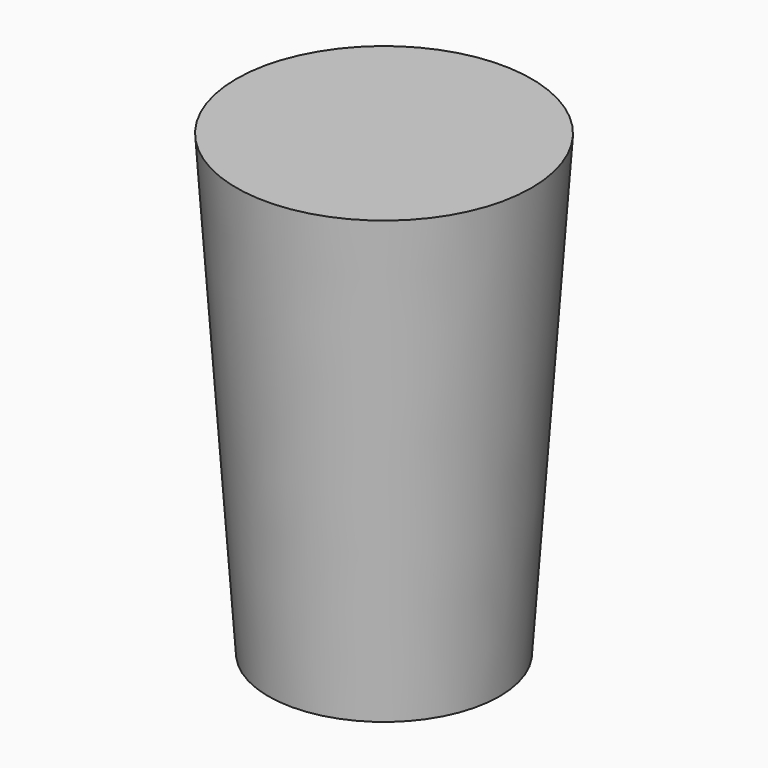
from build123d import *

# Parameters (mm, degrees)
F0_R     = 50.4693117614
F1_DEPTH = 200
F1_TAPER = -4


with BuildPart() as f1:
    # F0 (on Top) → F1 (new body)
    with BuildSketch(Plane.XY):
        Circle(F0_R)
    extrude(amount=F1_DEPTH, taper=F1_TAPER)


solid = f1.part
